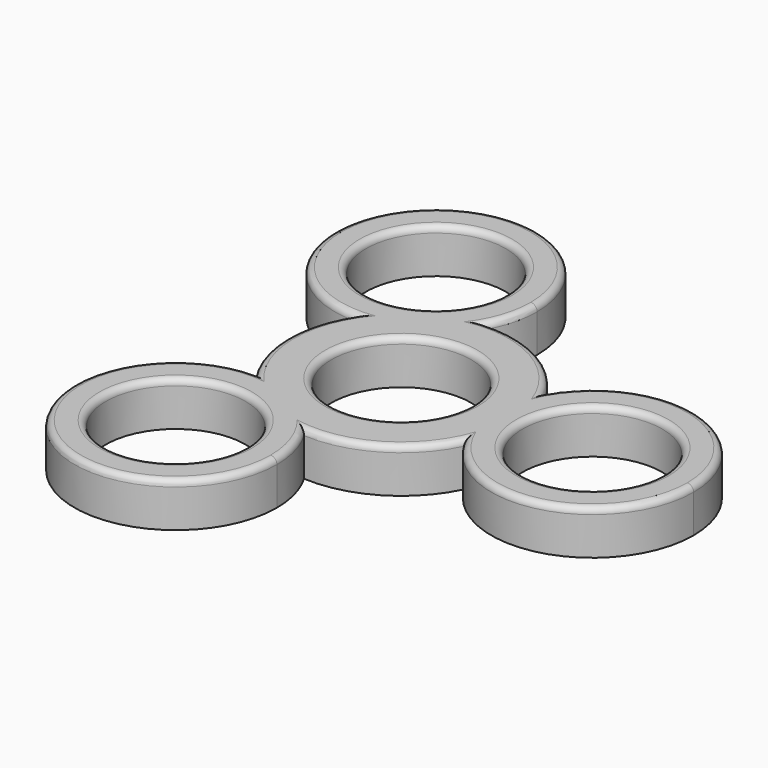
from build123d import *

# Parameters (mm, degrees)
F0_R     = 11.05
F1_DEPTH = 7
F2_R     = 1


# Not quite as in the source:
# - a feature names something its author has since deleted; it is built from what else it names


with BuildPart() as f1:
    # F0 (on Top) → F1 (new body)
    with BuildSketch(Plane.XY):
        with BuildLine():
            ThreePointArc((16.2000438734, -7.8459275105), (17.5442410739, -4.0248733073), (18, 0))
            ThreePointArc((18, 0), (17.5096912667, 4.1726144976), (16.0654764727, 8.1179101809))
            ThreePointArc((16.0654764727, 8.1179101809), (13.9995026295, 0.1180090099), (16.2000438734, -7.8459275105))
        make_face()
        with BuildLine():
            ThreePointArc((16.0654764727, 8.1179101809), (17.5096912667, 4.1726144976), (18, 0))
            ThreePointArc((18, 0), (17.5442410739, -4.0248733073), (16.2000438734, -7.8459275105))
            ThreePointArc((16.2000438734, -7.8459275105), (34.1952274917, -15.1870433254), (45.9989342061, 0.2528764497))
            ThreePointArc((45.9989342061, 0.2528764497), (34.064932009, 15.7276191574), (16.0654764727, 8.1179101809))
        make_face()
        with Locations((29.9989342061, 0.2528764497)):
            Circle(F0_R, mode=Mode.SUBTRACT)
        with BuildLine():
            ThreePointArc((16.2000438734, -7.8459275105), (13.9995026295, 0.1180090099), (16.0654764727, 8.1179101809))
            ThreePointArc((16.0654764727, 8.1179101809), (8.8682818041, 15.6637664003), (-1.3052493964, 17.952613292))
            ThreePointArc((-1.3052493964, 17.952613292), (-7.1019501152, 12.0649204126), (-15.0630546786, 9.8541556588))
            ThreePointArc((-15.0630546786, 9.8541556588), (-17.9993605237, -0.1517258698), (-14.894794477, -10.1066857815))
            ThreePointArc((-14.894794477, -10.1066857815), (-6.8975525143, -12.1829294224), (-1.0024217941, -17.9720658397))
            ThreePointArc((-1.0024217941, -17.9720658397), (9.1310787195, -15.5120405304), (16.2000438734, -7.8459275105))
        make_face()
        Circle(F0_R, mode=Mode.SUBTRACT)
        with BuildLine():
            ThreePointArc((-15.0630546786, 9.8541556588), (-7.1019501152, 12.0649204126), (-1.3052493964, 17.952613292))
            ThreePointArc((-1.3052493964, 17.952613292), (-9.1310787195, 15.5120405304), (-15.0630546786, 9.8541556588))
        make_face()
        with BuildLine():
            ThreePointArc((-15.0630546786, 9.8541556588), (-9.1310787195, 15.5120405304), (-1.3052493964, 17.952613292))
            ThreePointArc((-1.3052493964, 17.952613292), (0.2510448679, 21.7675375835), (0.7815354675, 25.8534008841))
            ThreePointArc((0.7815354675, 25.8534008841), (-26.5869859329, 37.1120296269), (-15.0630546786, 9.8541556588))
        make_face()
        with Locations((-15.2184645325, 25.8534008841)):
            Circle(F0_R, mode=Mode.SUBTRACT)
        with BuildLine():
            ThreePointArc((1.2195303265, -26.1062773338), (0.6540495297, -21.890163369), (-1.0024217941, -17.9720658397))
            ThreePointArc((-1.0024217941, -17.9720658397), (-8.8682818041, -15.6637664003), (-14.894794477, -10.1066857815))
            ThreePointArc((-14.894794477, -10.1066857815), (-26.0536857884, -37.4603338084), (1.2195303265, -26.1062773338))
        make_face()
        with Locations((-14.7804696735, -26.1062773338)):
            Circle(F0_R, mode=Mode.SUBTRACT)
        with BuildLine():
            ThreePointArc((-14.894794477, -10.1066857815), (-8.8682818041, -15.6637664003), (-1.0024217941, -17.9720658397))
            ThreePointArc((-1.0024217941, -17.9720658397), (-6.8975525143, -12.1829294224), (-14.894794477, -10.1066857815))
        make_face()
    extrude(amount=F1_DEPTH)

    # F2
    f2_edges = [f1.edges().sort_by_distance(p)[0] for p in [
        (45.998366, 0.387744, 7),
        (8.868282, 15.663766, 7),
        (-23.334979, 39.641881, 7),
        (-17.999361, -0.151726, 7),
        (-22.663387, -40.029625, 7),
        (9.131079, -15.512041, 7),
        (18.948934, 0.252876, 7),
        (-11.05, 0, 7),
        (-26.268465, 25.853401, 7),
        (-25.83047, -26.106277, 7),
    ]]
    fillet(f2_edges, radius=F2_R)


solid = f1.part
